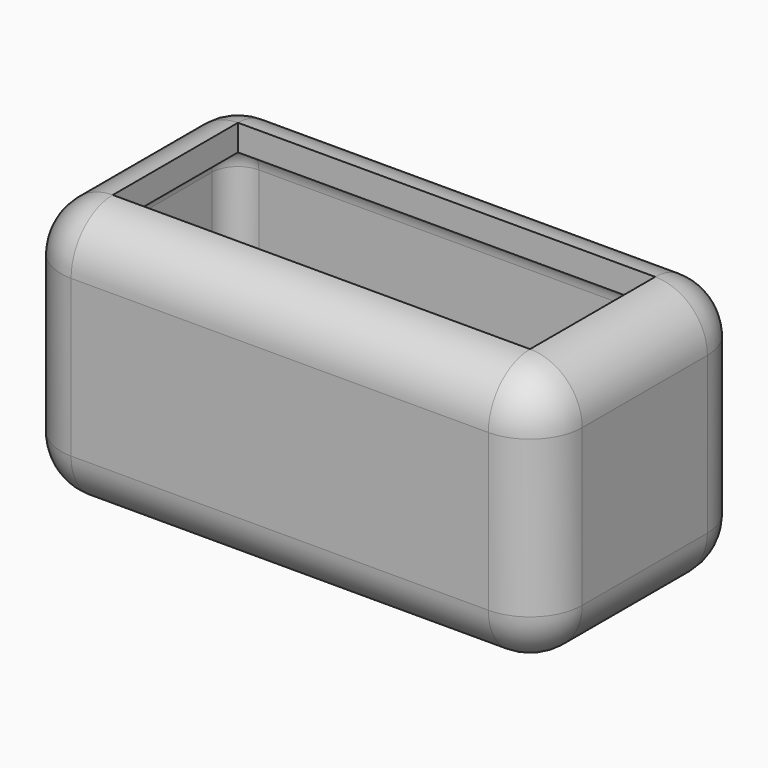
from build123d import *

# Parameters (mm, degrees)
F0_W     = 50
F0_H     = 25
F1_DEPTH = 25
F2_R     = 5
F3_T     = -2.5


# Not quite as in the source:
# - a shell that OpenCascade refuses in one call is made with other operations: the cavity is built on its own and cut out


with BuildPart() as f1:
    # F0 (on Top) → F1 (new body)
    with BuildSketch(Plane.XY):
        with Locations((-25, 12.5)):
            Rectangle(F0_W, F0_H)
    extrude(amount=F1_DEPTH)

    # F2
    f2_edges = [f1.edges().sort_by_distance(p)[0] for p in [
        (0, 12.5, 25),
        (-25, 0, 25),
        (-50, 12.5, 25),
        (-25, 25, 25),
        (-50, 25, 12.5),
        (-50, 12.5, 0),
        (-50, 0, 12.5),
        (-25, 0, 0),
        (0, 12.5, 0),
        (-25, 25, 0),
        (0, 25, 12.5),
        (0, 0, 12.5),
    ]]
    fillet(f2_edges, radius=F2_R)

    # F3: a shell. OpenCascade refuses it in one call, so the cavity is built on its own and cut out:
    # the body offset inwards by the wall thickness, plus a prism from it out through each open face.
    f3_core = offset(f1.part, amount=F3_T, mode=Mode.PRIVATE)
    f3_exits = [f3_core.faces().sort_by_distance(p)[0] for p in [
        (-25, 12.5, 22.5),
    ]]
    add(f3_core, mode=Mode.SUBTRACT)
    extrude(f3_exits, amount=-F3_T, mode=Mode.SUBTRACT)


solid = f1.part
